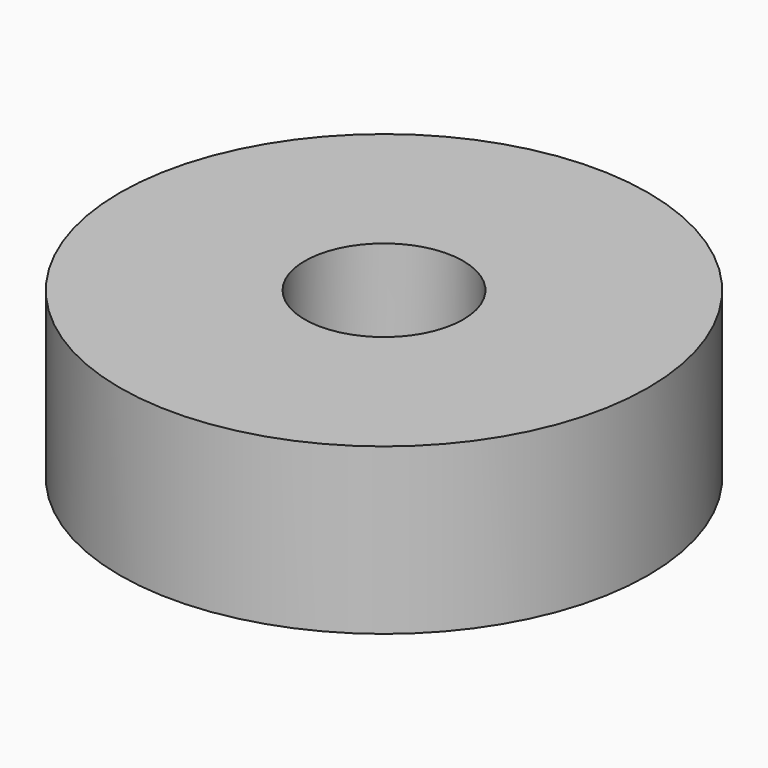
from build123d import *

# Parameters (mm, degrees)
F0_R     = 5.08
F0_R_2   = 1.524
F1_DEPTH = 3.175


# Not quite as in the source:
# - a length typed as a fraction of an inch, garbled in the dataset ("3 / 203.2 mm" for 3/8 in), is restored


with BuildPart() as f1:
    # F0 (on Top) → F1 (new body)
    with BuildSketch(Plane.XY):
        Circle(F0_R)
        Circle(F0_R_2, mode=Mode.SUBTRACT)
    extrude(amount=F1_DEPTH)


solid = f1.part
